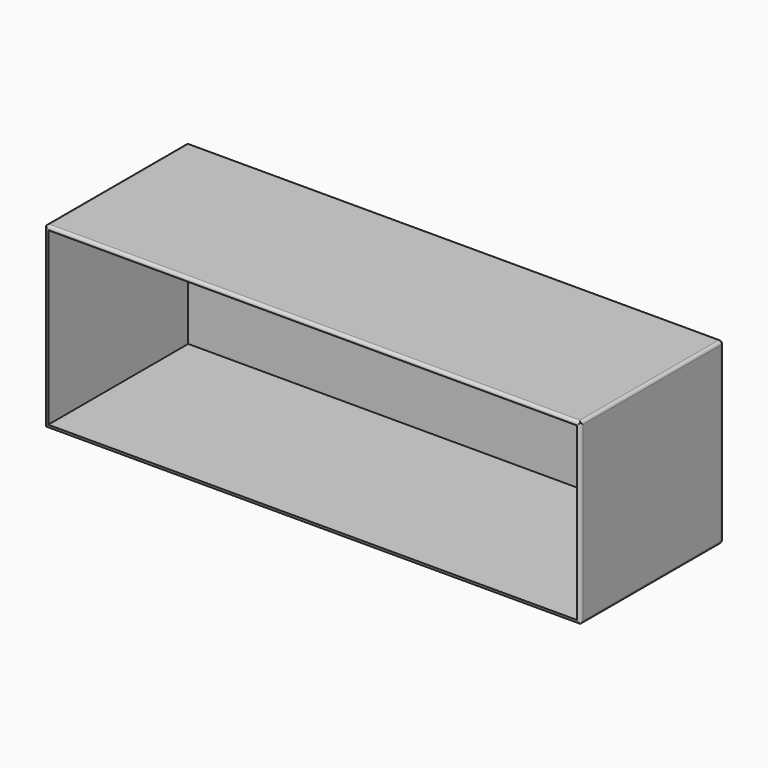
from build123d import *

# Parameters (mm, degrees)
F0_W         = 914.4
F0_H         = 304.8
F1_DEPTH     = 304.8
F2_T         = -6.35
F3_R         = 5.08
F4_T1_DEPTH  = 307.34
F4_T3_DEPTH  = 904.24
F4_T5_DEPTH  = 294.64
F4_S9_W      = 5.1816
F4_S9_H      = 5.1816
F4_T10_DEPTH = 5.1816
F4_S15_W     = 5.1816
F4_S15_H     = 5.1816
F4_T16_DEPTH = 5.1816
F4_S21_W     = 5.1816
F4_S21_H     = 5.1816
F4_T22_DEPTH = 5.1816
F4_S27_W     = 5.1816
F4_S27_H     = 5.1816
F4_T28_DEPTH = 5.1816


# Not quite as in the source:
# - a fillet or chamfer that OpenCascade refuses, or shapes differently, is made with other operations: its cross-section is extruded or revolved along the edge and cut away or added


with BuildPart() as f1:
    # F0 (on Front) → F1 (new body)
    with BuildSketch(Plane.XZ):
        with Locations((-4.9767009914, -156.8363738472)):
            Rectangle(F0_W, F0_H)
    extrude(amount=F1_DEPTH)

    # F2
    f2_openings = [f1.faces().sort_by_distance(p)[0] for p in [
        (-4.976701, -304.8, -156.836374),
    ]]
    offset(amount=F2_T, openings=f2_openings)

    # F3
    f3_edges = [f1.edges().sort_by_distance(p)[0] for p in [
        (-4.976701, -304.8, -4.436374),
        (-462.176701, -304.8, -156.836374),
        (-4.976701, -304.8, -309.236374),
        (452.223299, -304.8, -156.836374),
    ]]
    fillet(f3_edges, radius=F3_R)

    # F4: fillet of radius 5.08 on 12 edges, made by hand

    # F4_s2 → F4_t1 (cut)
    with BuildSketch(Plane.XZ.offset(5.08)):
        with BuildLine():
            ThreePointArc((452.2232990086, -9.5163738472), (450.735401457, -5.9242713988), (447.1432990086, -4.4363738472))
            Line((447.1432990086, -4.4363738472), (452.2232990086, -4.4363738472))
            Line((452.2232990086, -4.4363738472), (452.2232990086, -9.5163738472))
        make_face()
        with BuildLine():
            ThreePointArc((-457.0967009914, -4.4363738472), (-460.6888034398, -5.9242713988), (-462.1767009914, -9.5163738472))
            Line((-462.1767009914, -9.5163738472), (-462.1767009914, -4.4363738472))
            Line((-462.1767009914, -4.4363738472), (-457.0967009914, -4.4363738472))
        make_face()
        with BuildLine():
            ThreePointArc((-457.0967009914, -309.2363738472), (-460.6888034398, -307.7484762956), (-462.1767009914, -304.1563738472))
            Line((-462.1767009914, -304.1563738472), (-462.1767009914, -309.2363738472))
            Line((-462.1767009914, -309.2363738472), (-457.0967009914, -309.2363738472))
        make_face()
        with BuildLine():
            ThreePointArc((452.2232990086, -304.1563738472), (450.735401457, -307.7484762956), (447.1432990086, -309.2363738472))
            Line((447.1432990086, -309.2363738472), (452.2232990086, -309.2363738472))
            Line((452.2232990086, -309.2363738472), (452.2232990086, -304.1563738472))
        make_face()
    extrude(amount=F4_T1_DEPTH, mode=Mode.SUBTRACT)

    # F4_s4 → F4_t3 (cut)
    with BuildSketch(Plane.YZ.offset(-457.0967009914)):
        with BuildLine():
            ThreePointArc((0, -9.5163738472), (-1.4878975516, -5.9242713988), (-5.08, -4.4363738472))
            Line((-5.08, -4.4363738472), (0, -4.4363738472))
            Line((0, -4.4363738472), (0, -9.5163738472))
        make_face()
        with BuildLine():
            ThreePointArc((-5.08, -309.2363738472), (-1.4878975516, -307.7484762956), (0, -304.1563738472))
            Line((0, -304.1563738472), (0, -309.2363738472))
            Line((0, -309.2363738472), (-5.08, -309.2363738472))
        make_face()
    extrude(amount=F4_T3_DEPTH, mode=Mode.SUBTRACT)

    # F4_s6 → F4_t5 (cut)
    with BuildSketch(Plane.XY.offset(-304.1563738472)):
        with BuildLine():
            ThreePointArc((-457.0967009914, 0), (-460.6888034398, -1.4878975516), (-462.1767009914, -5.08))
            Line((-462.1767009914, -5.08), (-462.1767009914, 0))
            Line((-462.1767009914, 0), (-457.0967009914, 0))
        make_face()
        with BuildLine():
            ThreePointArc((452.2232990086, -5.08), (450.735401457, -1.4878975516), (447.1432990086, 0))
            Line((447.1432990086, 0), (452.2232990086, 0))
            Line((452.2232990086, 0), (452.2232990086, -5.08))
        make_face()
    extrude(amount=F4_T5_DEPTH, mode=Mode.SUBTRACT)


with BuildPart() as f4_tool8:
    # F4_s9 → F4_t10 (new body)
    with BuildSketch(Plane.YZ.offset(447.1432990086)):
        with Locations((-2.4892, -6.9255738472)):
            Rectangle(F4_S9_W, F4_S9_H)
    extrude(amount=F4_T10_DEPTH)

    # F4_s11 → F4_t12 (revolve, cut)
    with BuildSketch(Plane(origin=(447.1432990086, -5.08, -9.5163738472), x_dir=(0, -0.7071067812, -0.7071067812), z_dir=(0, -0.7071067812, 0.7071067812))):
        with BuildLine():
            ThreePointArc((0, -5.08), (5.08, 0), (0, 5.08))
            Line((0, 5.08), (0, -5.08))
        make_face()
    revolve(axis=Axis((447.1432990086, -5.08, -9.5163738472), (1, 0, 0)), mode=Mode.SUBTRACT)


with BuildPart() as f1_1:
    add(f1.part)

    # F4_t7: cut F4_tool8
    add(f4_tool8.part, mode=Mode.SUBTRACT)


with BuildPart() as f4_tool14:
    # F4_s15 → F4_t16 (new body)
    with BuildSketch(Plane.XZ.offset(5.08)):
        with Locations((-459.6875009914, -6.9255738472)):
            Rectangle(F4_S15_W, F4_S15_H)
    extrude(amount=-F4_T16_DEPTH)

    # F4_s17 → F4_t18 (revolve, cut)
    with BuildSketch(Plane(origin=(-457.0967009914, -5.08, -9.5163738472), x_dir=(0.7071067812, 0, -0.7071067812), z_dir=(0.7071067812, 0, 0.7071067812))):
        with BuildLine():
            ThreePointArc((0, -5.08), (5.08, 0), (0, 5.08))
            Line((0, 5.08), (0, -5.08))
        make_face()
    revolve(axis=Axis((-457.0967009914, -5.08, -9.5163738472), (0, 1, 0)), mode=Mode.SUBTRACT)


with BuildPart() as f1_2:
    add(f1_1.part)

    # F4_t13: cut F4_tool14
    add(f4_tool14.part, mode=Mode.SUBTRACT)


with BuildPart() as f4_tool20:
    # F4_s21 → F4_t22 (new body)
    with BuildSketch(Plane.XY.offset(-304.1563738472)):
        with Locations((-459.6875009914, -2.4892)):
            Rectangle(F4_S21_W, F4_S21_H)
    extrude(amount=-F4_T22_DEPTH)

    # F4_s23 → F4_t24 (revolve, cut)
    with BuildSketch(Plane(origin=(-457.0967009914, -5.08, -304.1563738472), x_dir=(0.7071067812, -0.7071067812, 0), z_dir=(0.7071067812, 0.7071067812, 0))):
        with BuildLine():
            ThreePointArc((0, -5.08), (5.08, 0), (0, 5.08))
            Line((0, 5.08), (0, -5.08))
        make_face()
    revolve(axis=Axis((-457.0967009914, -5.08, -304.1563738472), (0, 0, -1)), mode=Mode.SUBTRACT)


with BuildPart() as f1_3:
    add(f1_2.part)

    # F4_t19: cut F4_tool20
    add(f4_tool20.part, mode=Mode.SUBTRACT)


with BuildPart() as f4_tool26:
    # F4_s27 → F4_t28 (new body)
    with BuildSketch(Plane.YZ.offset(447.1432990086)):
        with Locations((-2.4892, -306.7471738472)):
            Rectangle(F4_S27_W, F4_S27_H)
    extrude(amount=F4_T28_DEPTH)

    # F4_s29 → F4_t30 (revolve, cut)
    with BuildSketch(Plane(origin=(447.1432990086, -5.08, -304.1563738472), x_dir=(0, -0.7071067812, 0.7071067812), z_dir=(0, 0.7071067812, 0.7071067812))):
        with BuildLine():
            ThreePointArc((0, -5.08), (5.08, 0), (0, 5.08))
            Line((0, 5.08), (0, -5.08))
        make_face()
    revolve(axis=Axis((447.1432990086, -5.08, -304.1563738472), (1, 0, 0)), mode=Mode.SUBTRACT)


with BuildPart() as f1_4:
    add(f1_3.part)

    # F4_t25: cut F4_tool26
    add(f4_tool26.part, mode=Mode.SUBTRACT)


solid = f1_4.part
